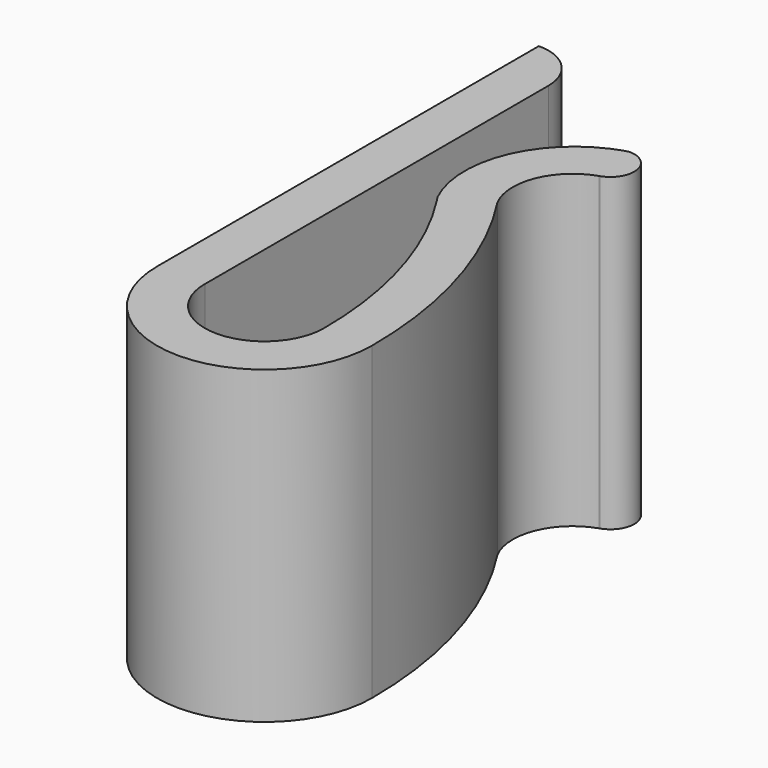
from build123d import *

# Parameters (mm, degrees)
F1_DEPTH = 13
F2_R     = 1.99999


# Not quite as in the source:
# - a fillet or chamfer is up to 0.001 mm smaller than in the source, because OpenCascade refuses the exact size


with BuildPart() as f1:
    # F0 (on Top) → F1 (new body)
    with BuildSketch(Plane.XY):
        with BuildLine():
            Line((0, 10), (0, 24.5))
            Line((0, 24.5), (-2, 24.5))
            Line((-2, 24.5), (-2, 4.5))
            ThreePointArc((-2, 4.5), (2.5, 0), (7, 4.5))
            ThreePointArc((7, 4.5), (6.2015841123, 9.9720743607), (3.8729089523, 14.9878831427))
            ThreePointArc((3.8729089523, 14.9878831427), (3.7530227087, 17.0940905495), (5.2871913605, 18.5421267712))
            ThreePointArc((5.2871913605, 18.5421267712), (5.3073257689, 18.5487259027), (5.3275153833, 18.5551541535))
            ThreePointArc((5.3275153833, 18.5551541535), (5.9849559235, 19.6728057544), (4.9863180052, 20.4999063971))
            ThreePointArc((4.9863180052, 20.4999063971), (4.6777817893, 20.4017930021), (4.3769319754, 20.2821676525))
            ThreePointArc((4.3769319754, 20.2821676525), (1.9143946428, 17.6625142897), (2.0963385188, 14.0717524929))
            ThreePointArc((2.0963385188, 14.0717524929), (2.172582587, 13.95665433), (2.2479018586, 13.8409488747))
            ThreePointArc((2.2479018586, 13.8409488747), (4.2976593275, 9.3689672945), (5, 4.5))
            ThreePointArc((5, 4.5), (2.5, 2), (0, 4.5))
            Line((0, 4.5), (0, 10))
        make_face()
    extrude(amount=F1_DEPTH)

    # F2 (radius 2 in the source; OpenCascade refuses exactly that, so slightly less here)
    f2_edges = [f1.edges().sort_by_distance(p)[0] for p in [
        (0, 24.5, 6.5),
    ]]
    fillet(f2_edges, radius=F2_R)


solid = f1.part
